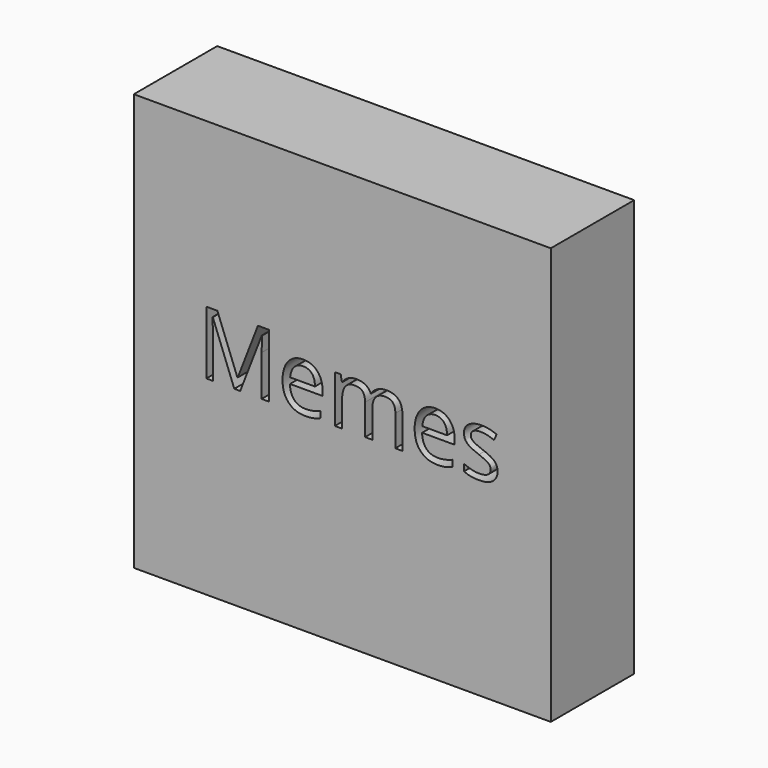
from build123d import *

# Parameters (mm, degrees)
F0_W         = 60
F0_H         = 60
F1_DEPTH     = 15
F2_TEXT_SIZE = 12.7467119859
F3_DEPTH     = 15


# Not quite as in the source:
# - Text() gives the source's letters only with a copy of the font that has no kerning and outlines rounded to 1/6400 em; it was checked with that copy


with BuildPart() as f1:
    # F0 (on Front) → F1 (new body)
    with BuildSketch(Plane.XZ):
        with Locations((-7.7467125654, 30)):
            Rectangle(F0_W, F0_H)
    extrude(amount=F1_DEPTH)

    # F2 (on face) → F3 (cut)
    with BuildSketch(Plane.XZ.offset(15)):
        with Locations((-28.5690770252, 27.3848697543)):
            Text('Memes', F2_TEXT_SIZE, font='Open Sans', text_align=(TextAlign.LEFT, TextAlign.BOTTOM))
    extrude(amount=-F3_DEPTH, mode=Mode.SUBTRACT)


solid = f1.part
